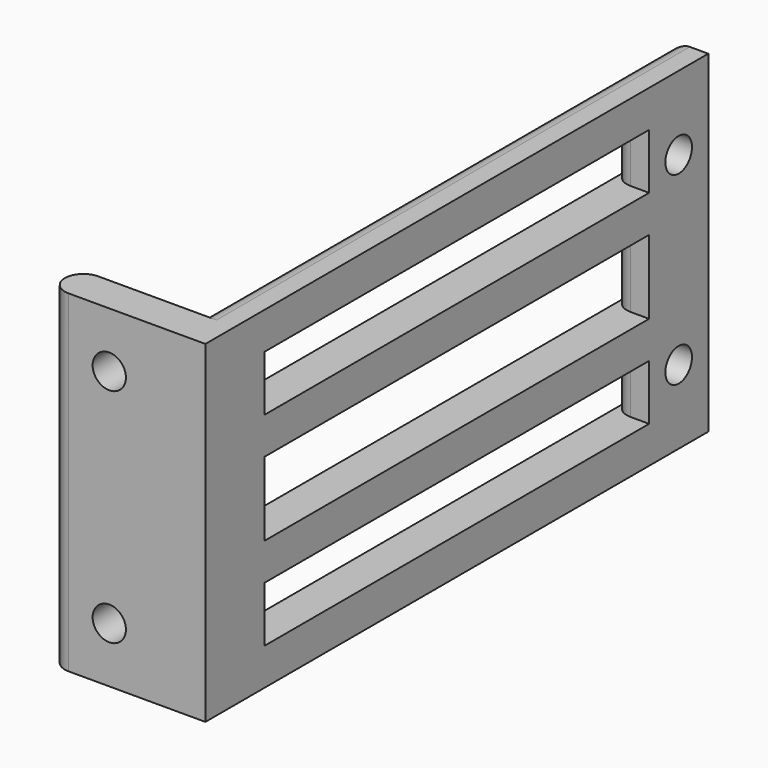
from build123d import *

# Parameters (mm, degrees)
F0_W     = 16
F0_H     = 5
F1_DEPTH = 45
F2_R     = 2.25
F3_DEPTH = 5
F4_W     = 65
F4_H     = 7.5
F4_R     = 2.25
F4_H_2   = 10
F5_DEPTH = 5
F6_R     = 2.49999


# Not quite as in the source:
# - a fillet or chamfer is up to 0.001 mm smaller than in the source, because OpenCascade refuses the exact size
# - a feature names something its author has since deleted; it is built from what else it names


with BuildPart() as f1:
    # F0 (on Top) → F1 (new body)
    with BuildSketch(Plane.XY):
        Polygon((-4.1043104958, 55.0339419188), (-4.1043104958, -24.9660580812), (-4.1043104958, -29.9660580812), (0.8956895042, -29.9660580812), (0.8956895042, 55.0339419188), align=None)
        with Locations((-12.1043104958, -27.4660580812)):
            Rectangle(F0_W, F0_H)
    extrude(amount=F1_DEPTH)

    # F2 (on face) → F3 (cut, through all)
    with BuildSketch(Plane(origin=(0, -24.9660580812, 0), x_dir=(-1, 0, 0), z_dir=(0, 1, 0))):
        with Locations((12.1043104958, 7.5)):
            Circle(F2_R)
        with Locations((12.1043104958, 37.5)):
            Circle(F2_R)
    extrude(amount=-F3_DEPTH, mode=Mode.SUBTRACT)

    # F4 (on face) → F5 (cut, through all)
    with BuildSketch(Plane(origin=(-4.1043104958, 0, 0), x_dir=(0, -1, 0), z_dir=(-1, 0, 0))):
        with Locations((-12.5339419188, 8.75)):
            Rectangle(F4_W, F4_H)
        with Locations((-50.0339419188, 35)):
            Circle(F4_R)
        with Locations((-50.0339419188, 10)):
            Circle(F4_R)
        with Locations((-12.5339419188, 22.5)):
            Rectangle(F4_W, F4_H_2)
        with Locations((-12.5339419188, 36.25)):
            Rectangle(F4_W, F4_H)
    extrude(amount=-F5_DEPTH, mode=Mode.SUBTRACT)

    # F6 (radius 2.5 in the source; OpenCascade refuses exactly that, so slightly less here)
    f6_edges = [f1.edges().sort_by_distance(p)[0] for p in [
        (-4.10431, 15.033942, 0),
        (-4.10431, 55.033942, 22.5),
        (-4.10431, 15.033942, 45),
        (-4.10431, 45.033942, 8.75),
        (-4.10431, 45.033942, 22.5),
        (-4.10431, 45.033942, 36.25),
        (-4.10431, -19.966058, 8.75),
        (-4.10431, -19.966058, 22.5),
        (-4.10431, -19.966058, 36.25),
        (-20.10431, -24.966058, 22.5),
        (-20.10431, -29.966058, 22.5),
    ]]
    fillet(f6_edges, radius=F6_R)


solid = f1.part
